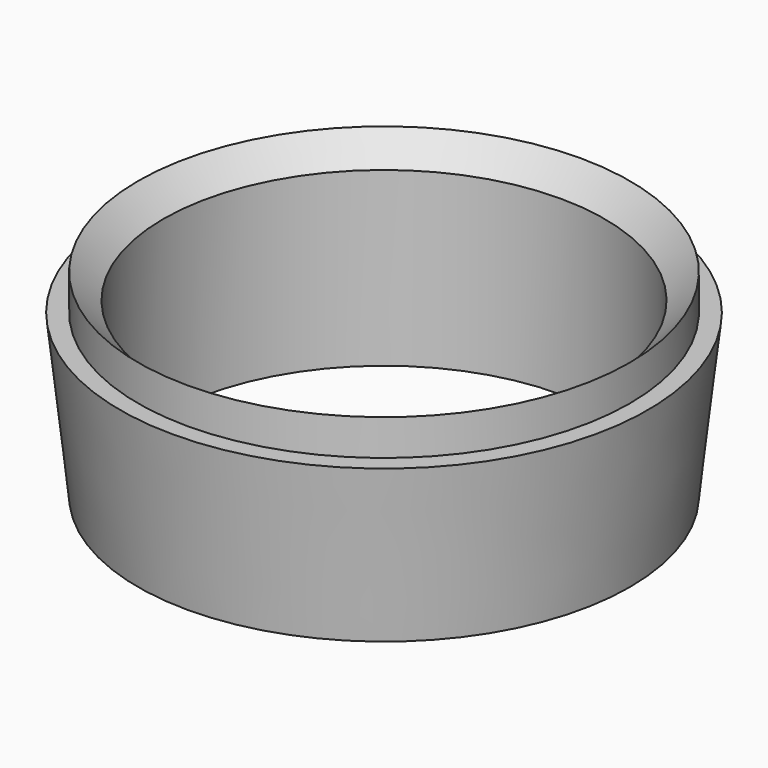
from build123d import *

# Parameters (mm, degrees)
F0_R     = 27.375
F0_R_2   = 24.565
F1_DEPTH = 22.09


# Not quite as in the source:
# - a fillet or chamfer that OpenCascade refuses, or shapes differently, is made with other operations: its cross-section is extruded or revolved along the edge and cut away or added


with BuildPart() as f1:
    # F0 (on Top) → F1 (new body)
    with BuildSketch(Plane.XY):
        Circle(F0_R)
        Circle(F0_R_2, mode=Mode.SUBTRACT)
    extrude(amount=F1_DEPTH)

    # F2: chamfer of 2.9 on 1 edges, made by hand

    # F2_s1 → F2_t2 (revolve, cut)
    with BuildSketch(Plane.XZ):
        Polygon((24.565, 19.19), (27.465, 22.09), (24.565, 22.09), align=None)
    revolve(axis=Axis((0, 0, 22.09), (0, 0, 1)), mode=Mode.SUBTRACT)


with BuildPart() as f5:
    # F3 (on Right) → F5 (revolve)
    with BuildSketch(Plane.YZ):
        Polygon((-29.375, 18), (-27.375, 0), (-27.375, 18), align=None)
    revolve(axis=Axis((0, 0, 7.8462371603), (0, 0, 1)))


solid = Compound([f1.part, f5.part])
